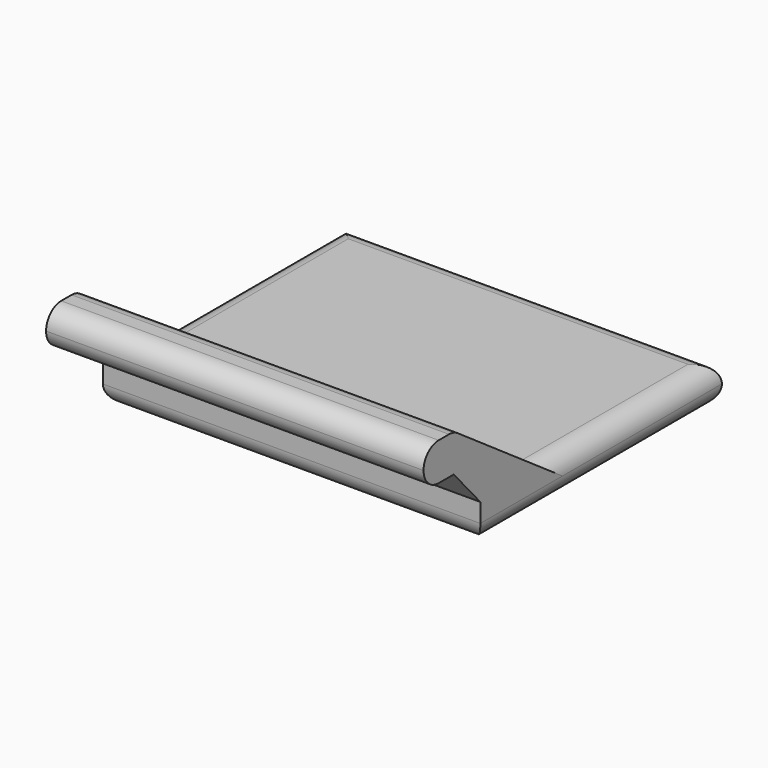
from build123d import *

# Parameters (mm, degrees)
F1_DEPTH = 25.4
F2_R     = 1.26999


# Not quite as in the source:
# - a fillet or chamfer is up to 0.001 mm smaller than in the source, because OpenCascade refuses the exact size


with BuildPart() as f1:
    # F0 (on Right) → F1 (new body)
    with BuildSketch(Plane.YZ):
        Polygon((14.605, 1.27), (-0.635, 1.27), (-7.9526191413, 6.35), (-10.4926191413, 6.35), (-10.4926191413, 3.81), (-7.9526191413, 3.81), (-5.715, 1.27), (-5.715, -1.27), (14.605, -1.27), align=None)
    extrude(amount=F1_DEPTH)

    # F2 (radius 1.27 in the source; OpenCascade refuses exactly that, so slightly less here)
    f2_edges = [f1.edges().sort_by_distance(p)[0] for p in [
        (12.7, -10.492619, 6.35),
        (12.7, -7.952619, 6.35),
        (12.7, -10.492619, 3.81),
        (12.7, 14.605, 1.27),
        (12.7, 14.605, -1.27),
        (12.7, -5.715, -1.27),
        (25.4, 6.985, 1.27),
        (0, 6.985, 1.27),
        (25.4, 4.445, -1.27),
        (0, 4.445, -1.27),
    ]]
    fillet(f2_edges, radius=F2_R)


solid = f1.part
